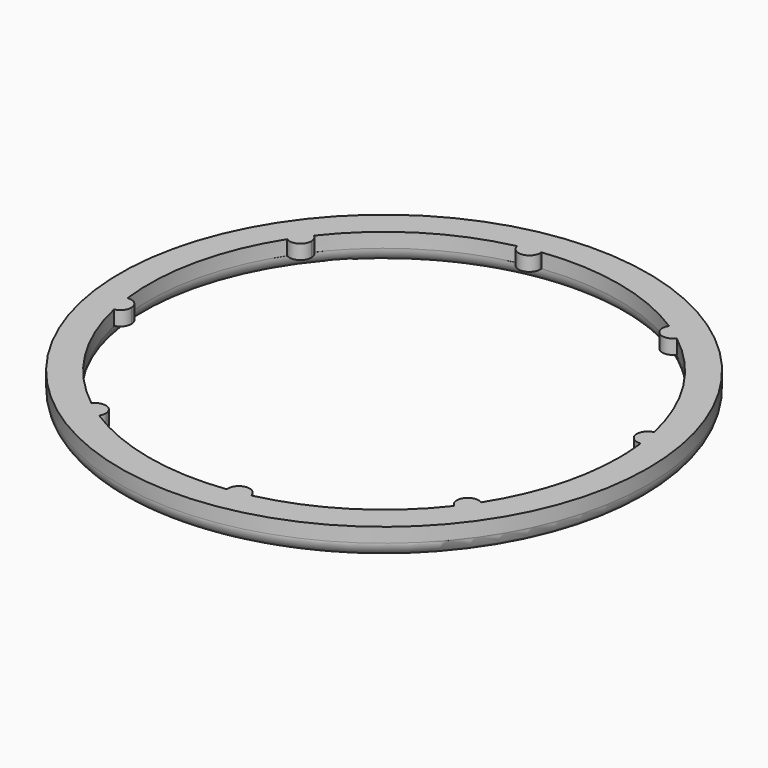
from build123d import *

# Parameters (mm, degrees)
F0_R     = 18.25
F0_R_2   = 16.25
F1_DEPTH = 2
F3_DEPTH = 1
F4_R     = 0.99999


# Not quite as in the source:
# - a fillet or chamfer is up to 0.001 mm smaller than in the source, because OpenCascade refuses the exact size


with BuildPart() as f1:
    # F0 (on Top) → F1 (new body)
    with BuildSketch(Plane.XY):
        Circle(F0_R)
        Circle(F0_R_2, mode=Mode.SUBTRACT)
    extrude(amount=F1_DEPTH)

    # F2 (on face) → F3 (join)
    with BuildSketch(Plane.XY.offset(2)):
        with BuildLine():
            ThreePointArc((-13.6956579083, 8.7459393126), (-12.9247475177, 8.70670819), (-12.5275195769, 9.368563064))
            ThreePointArc((-12.5275195769, 9.368563064), (-12.6077000662, 9.7059676033), (-12.8310977719, 9.9712301131))
            ThreePointArc((-12.8310977719, 9.9712301131), (-13.2775195769, 9.368563064), (-13.6956579083, 8.7459393126))
        make_face()
        with BuildLine():
            ThreePointArc((-13.6956579083, 8.7459393126), (-13.2775195769, 9.368563064), (-12.8310977719, 9.9712301131))
            ThreePointArc((-12.8310977719, 9.9712301131), (-13.8903281728, 9.8009582824), (-13.6956579083, 8.7459393126))
        make_face()
        with BuildLine():
            ThreePointArc((-2.0222318148, 16.1236806743), (-2.7640496576, 16.0131986027), (-3.4999795839, 15.8686055755))
            ThreePointArc((-3.4999795839, 15.8686055755), (-2.6914116674, 15.2667244087), (-2.0140496576, 16.0131986027))
            ThreePointArc((-2.0140496576, 16.0131986027), (-2.016097994, 16.0685909213), (-2.0222318148, 16.1236806743))
        make_face()
        with BuildLine():
            ThreePointArc((-2.0222318148, 16.1236806743), (-2.8916211803, 16.7522693075), (-3.4999795839, 15.8686055755))
            ThreePointArc((-3.4999795839, 15.8686055755), (-2.7640496576, 16.0131986027), (-2.0222318148, 16.1236806743))
        make_face()
        with BuildLine():
            ThreePointArc((-15.8686055755, -3.4999795839), (-16.0131986027, -2.7640496576), (-16.1236806743, -2.0222318148))
            ThreePointArc((-16.1236806743, -2.0222318148), (-16.7522693075, -2.8916211803), (-15.8686055755, -3.4999795839))
        make_face()
        with BuildLine():
            ThreePointArc((-15.2631986027, -2.7640496576), (-15.5234851935, -2.1959996802), (-16.1236806743, -2.0222318148))
            ThreePointArc((-16.1236806743, -2.0222318148), (-16.0131986027, -2.7640496576), (-15.8686055755, -3.4999795839))
            ThreePointArc((-15.8686055755, -3.4999795839), (-15.4339988227, -3.2405238067), (-15.2631986027, -2.7640496576))
        make_face()
        with BuildLine():
            ThreePointArc((9.9712301131, 12.8310977719), (9.368563064, 13.2775195769), (8.7459393126, 13.6956579083))
            ThreePointArc((8.7459393126, 13.6956579083), (8.9361678457, 12.664710981), (9.9712301131, 12.8310977719))
        make_face()
        with BuildLine():
            ThreePointArc((10.118563064, 13.2775195769), (9.5871176184, 13.9949691617), (8.7459393126, 13.6956579083))
            ThreePointArc((8.7459393126, 13.6956579083), (9.368563064, 13.2775195769), (9.9712301131, 12.8310977719))
            ThreePointArc((9.9712301131, 12.8310977719), (10.0807780199, 13.0424666965), (10.118563064, 13.2775195769))
        make_face()
        with BuildLine():
            ThreePointArc((-8.618563064, -13.2775195769), (-9.1335101836, -12.565304621), (-9.9712301131, -12.8310977719))
            ThreePointArc((-9.9712301131, -12.8310977719), (-9.368563064, -13.2775195769), (-8.7459393126, -13.6956579083))
            ThreePointArc((-8.7459393126, -13.6956579083), (-8.6511134792, -13.4960741312), (-8.618563064, -13.2775195769))
        make_face()
        with BuildLine():
            ThreePointArc((16.1236806743, 2.0222318148), (16.0131986027, 2.7640496576), (15.8686055755, 3.4999795839))
            ThreePointArc((15.8686055755, 3.4999795839), (15.274127898, 2.6364781349), (16.1236806743, 2.0222318148))
        make_face()
        with BuildLine():
            ThreePointArc((3.4999795839, -15.8686055755), (2.6364781349, -15.274127898), (2.0222318148, -16.1236806743))
            ThreePointArc((2.0222318148, -16.1236806743), (2.7640496576, -16.0131986027), (3.4999795839, -15.8686055755))
        make_face()
        with BuildLine():
            ThreePointArc((13.6956579083, -8.7459393126), (12.664710981, -8.9361678457), (12.8310977719, -9.9712301131))
            ThreePointArc((12.8310977719, -9.9712301131), (13.2775195769, -9.368563064), (13.6956579083, -8.7459393126))
        make_face()
    extrude(amount=-F3_DEPTH)

    # F4 (radius 1 in the source; OpenCascade refuses exactly that, so slightly less here)
    f4_edges = [f1.edges().sort_by_distance(p)[0] for p in [
        (-18.25, 0, 0),
        (-16.25, 0, 0),
    ]]
    fillet(f4_edges, radius=F4_R)


solid = f1.part
